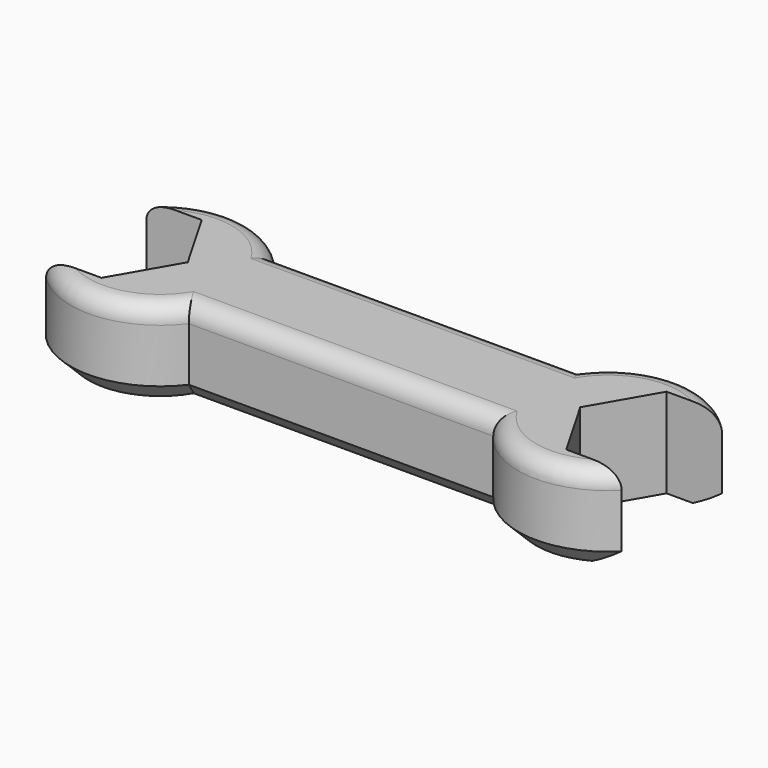
from build123d import *

# Parameters (mm, degrees)
F1_DEPTH = 6.35
F3_DEPTH = 12.701
F6_R     = 2.54
F7_SIZE  = 2.54


with BuildPart() as f1:
    # F0 (on Top) → F1 (new body, symmetric)
    with BuildSketch(Plane.XY):
        with BuildLine():
            Line((21.59, 7.62), (-21.59, 7.62))
            ThreePointArc((-21.59, 7.62), (-44.45, 0), (-21.59, -7.62))
            Line((-21.59, -7.62), (21.59, -7.62))
            ThreePointArc((21.59, -7.62), (44.45, 0), (21.59, 7.62))
        make_face()
    extrude(amount=F1_DEPTH, both=True)

    # F4: F3 across plane


with BuildPart() as f3:
    # F2 (on face) → F3 (new body, through all)
    with BuildSketch(Plane.XY.offset(6.35)):
        Polygon((-48.3652877862, 0), (-43.2326438931, -8.89), (-32.9673561069, -8.89), (-27.8347122138, 0), (-32.9673561069, 8.89), (-43.2326438931, 8.89), align=None)
    extrude(amount=-F3_DEPTH)


with BuildPart() as f1_1:
    add(f1.part)
    add(f3.part.mirror(Plane.YZ), mode=Mode.SUBTRACT)

    # F5: cut F3
    add(f3.part, mode=Mode.SUBTRACT)

    # F6
    f6_edges = [f1_1.edges().sort_by_distance(p)[0] for p in [
        (0, -7.62, 6.35),
        (-30.913065, -12.672393, 6.35),
        (-30.913065, 12.672393, 6.35),
        (0, 7.62, 6.35),
        (30.913065, 12.672393, 6.35),
        (30.913065, -12.672393, 6.35),
    ]]
    fillet(f6_edges, radius=F6_R)

    # F7
    f7_edges = [f1_1.edges().sort_by_distance(p)[0] for p in [
        (-30.913065, -12.672393, -6.35),
        (0, -7.62, -6.35),
        (30.913065, -12.672393, -6.35),
        (-30.913065, 12.672393, -6.35),
        (0, 7.62, -6.35),
        (30.913065, 12.672393, -6.35),
    ]]
    chamfer(f7_edges, length=F7_SIZE)


solid = f1_1.part
